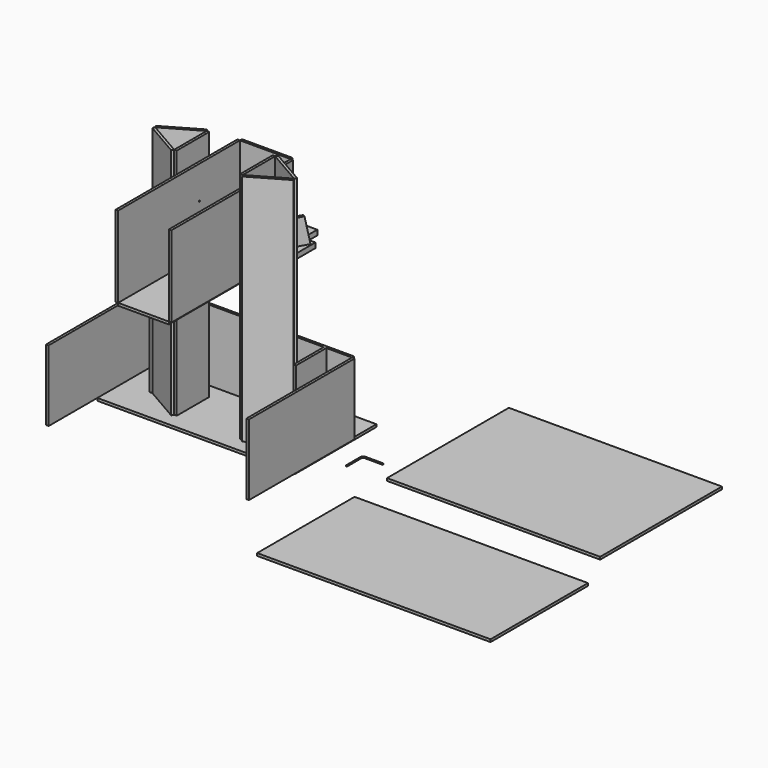
from build123d import *

# Parameters (mm, degrees)
F0_W      = 247.65
F0_H      = 88.9
F1_DEPTH  = 3.175
F2_W      = 3.175
F2_H      = 165.1
F3_DEPTH  = 88.9
F5_W      = 247.65
F5_H      = 3.175
F6_DEPTH  = 88.9
F7_W      = 3.175
F7_H      = 50.8
F8_DEPTH  = 292.1
F10_DEPTH = 292.1
F12_W     = 3.175
F12_H     = 47.199630657
F13_DEPTH = 88.9
F14_W     = 3.175
F14_H     = 47.199630657
F15_DEPTH = 88.9
F16_R     = 0.79375
F17_DEPTH = 50.8
F19_W     = 63.5
F19_H     = 190.5
F20_DEPTH = 3.175
F21_W     = 3.175
F21_H     = 190.5
F22_DEPTH = 101.6
F23_W     = 63.5
F23_H     = 101.6
F24_DEPTH = 3.175
F25_R     = 0.79375
F26_DEPTH = 161.926
F28_R     = 0.79375
F30_R     = 0.79375
F31_DEPTH = 31.75
F34_DEPTH = 6.35
F36_DEPTH = 31.75
F38_DEPTH = 205.8437401503
F39_W     = 266.7
F39_H     = 190.5
F40_DEPTH = 3.175
F41_W     = 292.1
F41_H     = 152.4
F42_DEPTH = 3.175
F43_W     = 247.65
F43_H     = 3.175
F44_DEPTH = 38.1


with BuildPart() as f1:
    # F0 (on Top) → F1 (new body)
    with BuildSketch(Plane.XY):
        Rectangle(F0_W, F0_H)
    extrude(amount=F1_DEPTH)

    # F43 (on face) → F44 (join)
    with BuildSketch(Plane(origin=(0, 44.45, 0), x_dir=(-1, 0, 0), z_dir=(0, 1, 0))):
        with Locations((0, 1.5875)):
            Rectangle(F43_W, F43_H)
    extrude(amount=F44_DEPTH)


with BuildPart() as f3:
    # F2 (on face) → F3 (new body)
    with BuildSketch(Plane.XY.offset(3.175)):
        with Locations((-125.4125, -38.1)):
            Rectangle(F2_W, F2_H)
    extrude(amount=F3_DEPTH)


with BuildPart() as f4_1:
    # F4: instance of F3
    add(f3.part.mirror(Plane.YZ))


with BuildPart() as f6:
    # F5 (on face) → F6 (new body, through all)
    with BuildSketch(Plane.XY.offset(3.175)):
        with Locations((0, 46.0375)):
            Rectangle(F5_W, F5_H)
    extrude(amount=F6_DEPTH)


with BuildPart() as f8:
    # F7 (on face) → F8 (new body)
    with BuildSketch(Plane.XY.offset(3.175)):
        with Locations((-41.275, 0)):
            Rectangle(F7_W, F7_H)
    extrude(amount=F8_DEPTH)


with BuildPart() as f10:
    # F9 (on face) → F10 (new body, through all)
    with BuildSketch(Plane.XY.offset(3.175)):
        Polygon((-42.8625, -25.4), (-86.8565905122, 0), (-88.4440905122, -2.749630657), (-44.45, -28.149630657), align=None)
    extrude(amount=F10_DEPTH)


with BuildPart() as f10b:
    # F9 (on face) → F10, piece 2 (new body, through all)
    with BuildSketch(Plane.XY.offset(3.175)):
        Polygon((-44.45, 28.149630657), (-88.4440905122, 2.749630657), (-86.8565905122, 0), (-42.8625, 25.4), align=None)
    extrude(amount=F10_DEPTH)


with BuildPart() as f11_1:
    # F11: instance of F10
    add(f10.part.mirror(Plane.YZ))


with BuildPart() as f11_2:
    # F11: instance of F10b
    add(f10b.part.mirror(Plane.YZ))


with BuildPart() as f11_3:
    # F11: instance of F8
    add(f8.part.mirror(Plane.YZ))


with BuildPart() as f13:
    # F12 (on face) → F13 (new body, through all)
    with BuildSketch(Plane.XY.offset(3.175)):
        with Locations((-90.0315905122, 20.8501846715)):
            Rectangle(F12_W, F12_H)
    extrude(amount=F13_DEPTH)


with BuildPart() as f15:
    # F14 (on face) → F15 (new body, through all)
    with BuildSketch(Plane.XY.offset(3.175)):
        with Locations((90.0315905122, 20.8501846715)):
            Rectangle(F14_W, F14_H)
    extrude(amount=F15_DEPTH)


with BuildPart() as f17_tool:
    # F16 (on Right) → F17 (new body, symmetric)
    with BuildSketch(Plane.YZ):
        with Locations((0, 231.775)):
            Circle(F16_R)
    extrude(amount=F17_DEPTH, both=True)


with BuildPart() as f8_1:
    add(f8.part)

    # F17: cut by f17_tool
    add(f17_tool.part, mode=Mode.SUBTRACT)


with BuildPart() as f11_3_1:
    add(f11_3.part)

    # F17: cut by f17_tool
    add(f17_tool.part, mode=Mode.SUBTRACT)


with BuildPart() as f20:
    # F19 (on offset) → F20 (new body)
    with BuildSketch(Plane.XY.offset(168.275)):
        with Locations((0, -31.75)):
            Rectangle(F19_W, F19_H)
    extrude(amount=F20_DEPTH)


with BuildPart() as f22:
    # F21 (on face) → F22 (new body)
    with BuildSketch(Plane.XY.offset(171.45)):
        with Locations((-33.3375, -31.75)):
            Rectangle(F21_W, F21_H)
    extrude(amount=F22_DEPTH)


with BuildPart() as f22b:
    # F21 (on face) → F22, piece 2 (new body)
    with BuildSketch(Plane.XY.offset(171.45)):
        with Locations((33.3375, -31.75)):
            Rectangle(F21_W, F21_H)
    extrude(amount=F22_DEPTH)


with BuildPart() as f24:
    # F23 (on face) → F24 (new body)
    with BuildSketch(Plane(origin=(0, 63.5, 0), x_dir=(-1, 0, 0), z_dir=(0, 1, 0))):
        with Locations((0, 222.25)):
            Rectangle(F23_W, F23_H)
    extrude(amount=F24_DEPTH)


with BuildPart() as f26_tool:
    # F25 (on face) → F26 (new body, through all)
    with BuildSketch(Plane.YZ.offset(34.925)):
        with Locations((0, 231.775)):
            Circle(F25_R)
    extrude(amount=-F26_DEPTH)


with BuildPart() as f22_1:
    add(f22.part)

    # F26: cut by f26_tool
    add(f26_tool.part, mode=Mode.SUBTRACT)


with BuildPart() as f22b_1:
    add(f22b.part)

    # F26: cut by f26_tool
    add(f26_tool.part, mode=Mode.SUBTRACT)


with BuildPart() as f29:
    # F29: sweep along a path in F27
    with BuildLine(Plane.XY) as f29_path:
        Line((152.4, 0), (152.4, 22.225))
        ThreePointArc((152.4, 22.225), (153.3299359697, 24.4700640303), (155.575, 25.4))
        Line((155.575, 25.4), (177.8, 25.4))
    # F28 (on Front) → F29 (sweep)
    with BuildSketch(Plane.XZ):
        with Locations((152.4, 0)):
            Circle(F28_R)
    sweep(path=f29_path.line)


with BuildPart() as f31:
    # F30 (on face) → F31 (new body)
    with BuildSketch(Plane(origin=(0, 63.5, 0), x_dir=(-1, 0, 0), z_dir=(0, 1, 0))):
        with Locations((-35.71875, 257.175)):
            Circle(F30_R)
    extrude(amount=-F31_DEPTH)


with BuildPart() as f34:
    # F33 (on offset) → F34 (new body)
    with BuildSketch(Plane.XY.offset(206.375)):
        Polygon((44.45, 28.149630657), (88.4440905122, 2.749630657), (88.4440905122, 31.324630657), (73.025, 31.324630657), (73.025, 53.549630657), (44.45, 53.549630657), align=None)
    extrude(amount=F34_DEPTH)


with BuildPart() as f36:
    # F35 (on face) → F36 (new body)
    with BuildSketch(Plane.XY.offset(212.725)):
        Polygon((74.6959372272, 10.687130657), (77.4455678842, 9.099630657), (86.9705678842, 25.5974145991), (84.2209372272, 27.1849145991), align=None)
    extrude(amount=F36_DEPTH)

    # F37 (on face) → F38 (cut, through all)
    with BuildSketch(Plane(origin=(54.1439202561, -31.2600069349, 0), x_dir=(0.5, 0.8660254038, 0), z_dir=(0.8660254038, -0.5, 0))):
        Polygon((65.6532952561, 244.475), (59.3032952561, 244.475), (65.6532952561, 212.725), align=None)
    extrude(amount=-F38_DEPTH, mode=Mode.SUBTRACT)


with BuildPart() as f40:
    # F39 (on Top) → F40 (new body)
    with BuildSketch(Plane.XY):
        with Locations((336.55, 95.25)):
            Rectangle(F39_W, F39_H)
    extrude(amount=F40_DEPTH)


with BuildPart() as f42:
    # F41 (on Top) → F42 (new body)
    with BuildSketch(Plane.XY):
        with Locations((349.25, -127)):
            Rectangle(F41_W, F41_H)
    extrude(amount=F42_DEPTH)


solid = Compound([f1.part, f3.part, f4_1.part, f6.part, f10.part, f10b.part, f11_1.part, f11_2.part, f13.part, f15.part, f8_1.part, f11_3_1.part, f20.part, f24.part, f22_1.part, f22b_1.part, f29.part, f31.part, f34.part, f36.part, f40.part, f42.part])
